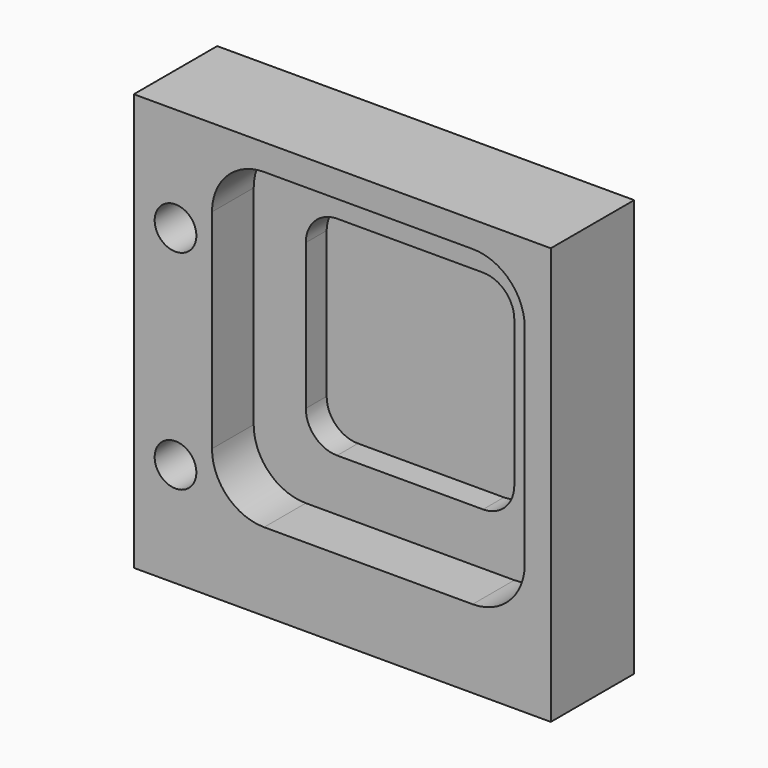
from build123d import *

# Parameters (mm, degrees)
F0_W     = 80
F0_H     = 80
F1_DEPTH = 20
F3_D     = 8
F3_DEPTH = 15
F3_TIP   = 2.4034424761
F5_DEPTH = 10
F6_DEPTH = 15


with BuildPart() as f1:
    # F0 (on Front) → F1 (new body)
    with BuildSketch(Plane.XZ):
        Rectangle(F0_W, F0_H)
    extrude(amount=F1_DEPTH)

    # F3
    with Locations(Plane.XZ.offset(20)):
        with Locations((-32, 20), (-32, -20)):
            Hole(F3_D / 2, depth=F3_DEPTH)
            with Locations((0, 0, -(F3_DEPTH + F3_TIP / 2))):  # 118° drill point
                Cone(0, F3_D / 2, F3_TIP, mode=Mode.SUBTRACT)

    # F4 (on face) → F5 (cut)
    with BuildSketch(Plane.XZ.offset(20)):
        with BuildLine():
            Line((25, 35), (-15, 35))
            ThreePointArc((-15, 35), (-22.0710678119, 32.0710678119), (-25, 25))
            Line((-25, 25), (-25, -15))
            ThreePointArc((-25, -15), (-22.0710678119, -22.0710678119), (-15, -25))
            Line((-15, -25), (25, -25))
            ThreePointArc((25, -25), (32.0710678119, -22.0710678119), (35, -15))
            Line((35, -15), (35, 25))
            ThreePointArc((35, 25), (32.0710678119, 32.0710678119), (25, 35))
        make_face()
        with BuildLine():
            ThreePointArc((-15, 19), (-13.2426406871, 23.2426406871), (-9, 25))
            Line((-9, 25), (19, 25))
            ThreePointArc((19, 25), (23.2426406871, 23.2426406871), (25, 19))
            Line((25, 19), (25, -9))
            ThreePointArc((25, -9), (23.2426406871, -13.2426406871), (19, -15))
            Line((19, -15), (-9, -15))
            ThreePointArc((-9, -15), (-13.2426406871, -13.2426406871), (-15, -9))
            Line((-15, -9), (-15, 19))
        make_face(mode=Mode.SUBTRACT)
    extrude(amount=-F5_DEPTH, mode=Mode.SUBTRACT)

    # F6 (cut): a face of the model
    f6_faces = [f1.faces().sort_by_distance(p)[0] for p in [
        (5, -20, 5),
    ]]
    extrude(f6_faces, amount=-F6_DEPTH, mode=Mode.SUBTRACT)


solid = f1.part
